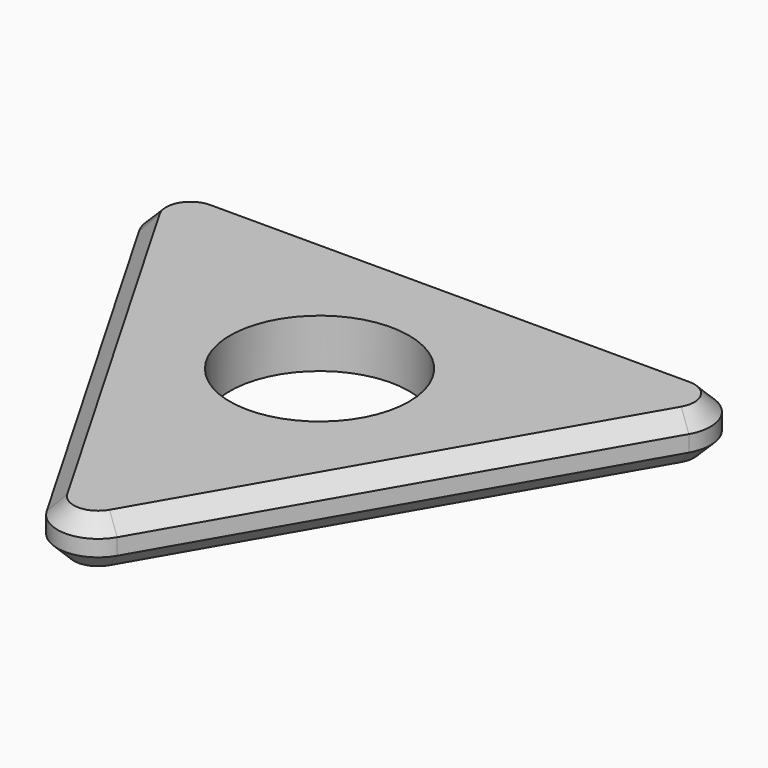
from build123d import *

# Parameters (mm, degrees)
F0_R     = 11
F1_DEPTH = 6
F2_SIZE  = 2


# Not quite as in the source:
# - a feature of the source that left no trace in its solid (it failed there, or was rolled back) is left out


with BuildPart() as f1:
    # F0 (on Top) → F1 (new body)
    with BuildSketch(Plane.XY):
        with BuildLine():
            Line((29.4397459622, 21.9970452561), (-29.4397459622, 21.9970452561))
            ThreePointArc((-29.4397459622, 21.9970452561), (-33.7698729811, 19.4970452561), (-33.7698729811, 14.4970452561))
            Line((-33.7698729811, 14.4970452561), (-4.3301270189, -36.4940905122))
            ThreePointArc((-4.3301270189, -36.4940905122), (0, -38.9940905122), (4.3301270189, -36.4940905122))
            Line((4.3301270189, -36.4940905122), (33.7698729811, 14.4970452561))
            ThreePointArc((33.7698729811, 14.4970452561), (33.7698729811, 19.4970452561), (29.4397459622, 21.9970452561))
        make_face()
        Circle(F0_R, mode=Mode.SUBTRACT)
    extrude(amount=F1_DEPTH)

    # F2
    f2_edges = [f1.edges().sort_by_distance(p)[0] for p in [
        (-19.05, -10.998523, 6),
        (-19.05, -10.998523, 0),
        (0, 21.997045, 6),
        (33.769873, 19.497045, 0),
        (33.769873, 19.497045, 6),
        (0, 21.997045, 0),
        (-33.769873, 19.497045, 0),
        (-33.769873, 19.497045, 6),
        (0, -38.994091, 0),
        (0, -38.994091, 6),
        (19.05, -10.998523, 0),
        (19.05, -10.998523, 6),
    ]]
    chamfer(f2_edges, length=F2_SIZE)


solid = f1.part
